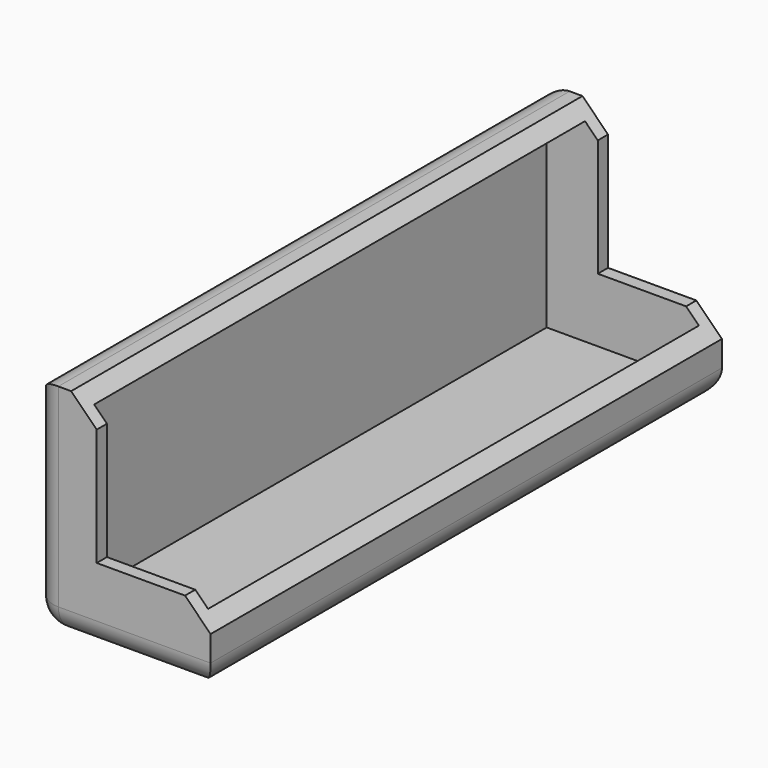
from build123d import *

# Parameters (mm, degrees)
F0_W        = 22.6290904153
F0_H        = 15.2400004526
F1_DEPTH    = 127
F2_T        = -2.54
F3_R        = 5.08
F4_T1_DEPTH = 153.1282991577


# Not quite as in the source:
# - a fillet or chamfer that OpenCascade refuses, or shapes differently, is made with other operations: its cross-section is extruded or revolved along the edge and cut away or added


with BuildPart() as f1:
    # F0 (on Front) → F1 (new body)
    with BuildSketch(Plane.XZ):
        Polygon((-22.6290904153, 0), (-22.6290904153, 15.2400004526), (-22.6290904153, 43.6418191694), (-35.3290904153, 43.6418191694), (-35.3290904153, 0), align=None)
        with Locations((-11.3145452077, 7.6200002263)):
            Rectangle(F0_W, F0_H)
    extrude(amount=F1_DEPTH)

    # F2
    f2_openings = [f1.faces().sort_by_distance(p)[0] for p in [
        (-22.62909, -63.5, 29.44091),
        (-11.314545, -63.5, 15.24),
    ]]
    offset(amount=F2_T, openings=f2_openings)

    # F3
    f3_edges = [f1.edges().sort_by_distance(p)[0] for p in [
        (-35.32909, -63.5, 43.641819),
        (0, -63.5, 0),
        (-35.32909, -63.5, 0),
        (-35.32909, 0, 21.82091),
        (-35.32909, -127, 21.82091),
        (-17.664545, -127, 0),
        (-17.664545, 0, 0),
    ]]
    fillet(f3_edges, radius=F3_R)

    # F4: chamfer of 5.08 on 2 edges, made by hand

    # F4_s2 → F4_t1 (cut)
    with BuildSketch(Plane.XZ.offset(-13.0641495789)):
        Polygon((-27.7090904153, 43.6418191694), (-22.6290904153, 38.5618191694), (-22.6290904153, 43.6418191694), align=None)
        Polygon((-5.08, 15.2400004526), (0, 10.1600004526), (0, 15.2400004526), align=None)
    extrude(amount=F4_T1_DEPTH, mode=Mode.SUBTRACT)


solid = f1.part
